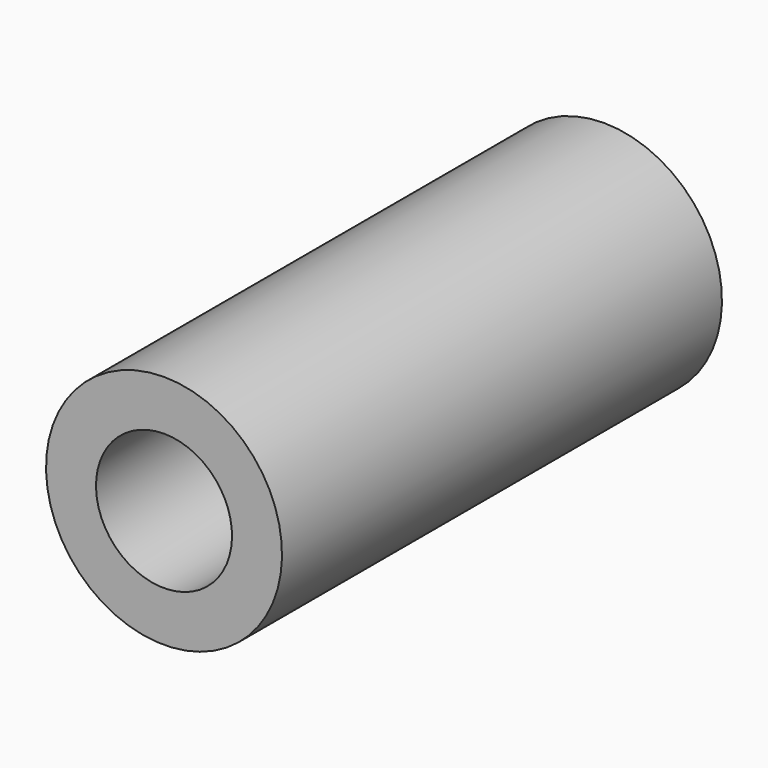
from build123d import *

# Parameters (mm, degrees)
F2_SIZE = 0.09999


# Not quite as in the source:
# - a fillet or chamfer is up to 0.001 mm smaller than in the source, because OpenCascade refuses the exact size


with BuildPart() as f1:
    # F0 (on Right) → F1 (revolve)
    with BuildSketch(Plane.YZ):
        with BuildLine():
            ThreePointArc((7.5617104388, 2.8), (8.3591026496, 4.0638625595), (9.425, 5.1112620751))
            Line((9.425, 5.1112620751), (9.425, 5.9))
            Line((9.425, 5.9), (-18.075, 5.9))
            Line((-18.075, 5.9), (-18.075, 3.4))
            Line((-18.075, 3.4), (-7.075, 3.4))
            Line((-7.075, 3.4), (-7.075, 3.3))
            Line((-7.075, 3.3), (-6.425, 3.3))
            Line((-6.425, 3.3), (6.425, 3.3))
            Line((6.425, 3.3), (6.925, 3.3))
            Line((6.925, 3.3), (6.925, 2.8))
            Line((6.925, 2.8), (7.5617104388, 2.8))
        make_face()
        Polygon((6.425, 3.3), (6.925, 2.8), (6.925, 3.3), align=None)
    revolve(axis=Axis((0, 1.2174843578, 0), (0, 1, 0)))

    # F2 (size 0.1 in the source; OpenCascade refuses exactly that, so slightly less here)
    f2_edges = [f1.edges().sort_by_distance(p)[0] for p in [
        (0, -7.075, -3.4),
    ]]
    chamfer(f2_edges, length=F2_SIZE)


solid = f1.part
